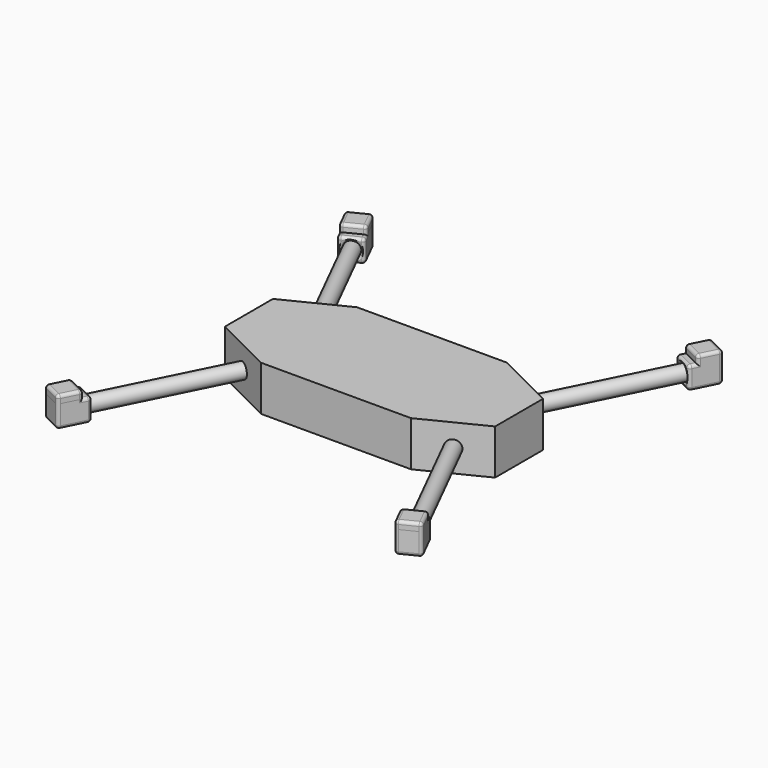
from build123d import *

# Parameters (mm, degrees)
F1_DEPTH      = 38.1
F2_R          = 6.35
F3_DEPTH      = 127
F4_W          = 19.05
F4_H          = 19.05
F5_DEPTH      = 12.7
F7_DEPTH      = 6.35
F9_T1_DEPTH   = 3.81
F9_T3_DEPTH   = 13.97
F9_T5_DEPTH   = 20.32
F9_T7_DEPTH   = 20.32
F9_T9_DEPTH   = 13.97
F9_T11_DEPTH  = 3.81
F9_T13_DEPTH  = 13.97
F9_T15_DEPTH  = 13.97
F9_T17_DEPTH  = 13.97
F9_S21_W      = 2.5908
F9_S21_H      = 2.5908
F9_T22_DEPTH  = 2.5908
F9_S27_W      = 2.5908
F9_S27_H      = 2.5908
F9_T28_DEPTH  = 2.5908
F9_S33_W      = 2.5908
F9_S33_H      = 2.5908
F9_T34_DEPTH  = 2.5908
F9_T40_DEPTH  = 2.5908
F9_S45_W      = 2.5908
F9_S45_H      = 2.5908
F9_T46_DEPTH  = 2.5908
F9_S51_W      = 2.5908
F9_S51_H      = 2.5908
F9_T52_DEPTH  = 2.5908
F9_S57_W      = 2.5908
F9_S57_H      = 2.5908
F9_T58_DEPTH  = 2.5908
F9_S63_W      = 2.5908
F9_S63_H      = 2.5908
F9_T64_DEPTH  = 2.5908
F9_S69_W      = 2.5908
F9_S69_H      = 2.5908
F9_T70_DEPTH  = 2.5908
F9_S75_W      = 2.5908
F9_S75_H      = 2.5908
F9_T76_DEPTH  = 2.5908
F9_T85_DEPTH  = 10.16
F9_T89_DEPTH  = 10.16
F9_T96_DEPTH  = 10.16
F9_T100_DEPTH = 10.16


# Not quite as in the source:
# - a fillet or chamfer that OpenCascade refuses, or shapes differently, is made with other operations: its cross-section is extruded or revolved along the edge and cut away or added


with BuildPart() as f1:
    # F0 (on Top) → F1 (new body)
    with BuildSketch(Plane.XY):
        Polygon((-63.5, 50.8), (-114.3, 25.4), (-114.3, -25.4), (-63.5, -50.8), (63.5, -50.8), (114.3, -25.4), (114.3, 25.4), (63.5, 50.8), align=None)
    extrude(amount=F1_DEPTH)


with BuildPart() as f3:
    # F2 (on face) → F3 (new body)
    with BuildSketch(Plane(origin=(-33.02, -66.04, 0), x_dir=(0.894427191, -0.4472135955, 0), z_dir=(-0.4472135955, -0.894427191, 0))):
        with Locations((-62.4757392913, 19.05)):
            Circle(F2_R)
    extrude(amount=F3_DEPTH)


with BuildPart() as f5:
    # F4 (on face) → F5 (new body, symmetric)
    with BuildSketch(Plane(origin=(-89.8161266285, -179.632253257, 0), x_dir=(0.894427191, -0.4472135955, 0), z_dir=(-0.4472135955, -0.894427191, 0))):
        with Locations((-62.4757392913, 19.05)):
            Rectangle(F4_W, F4_H)
    extrude(amount=F5_DEPTH, both=True)

    # F6 (on face) → F7 (join)
    with BuildSketch(Plane.XY.offset(28.575)):
        Polygon((-151.3757392913, -141.752931097), (-159.8951582856, -158.7917690856), (-142.8563202971, -167.3111880798), (-134.3369013028, -150.2723500913), align=None)
    extrude(amount=F7_DEPTH)

    # F8: cut F3
    add(f3.part, mode=Mode.SUBTRACT)

    # F9: fillet of radius 2.54 on 18 edges, made by hand

    # F9_s2 → F9_t1 (cut)
    with BuildSketch(Plane(origin=(-85.2724364982, -170.5448729964, 0), x_dir=(0, 0, 1), z_dir=(-0.4472135955, -0.894427191, 0))):
        with BuildLine():
            ThreePointArc((28.575, 69.4607392913), (27.8310512242, 71.2567905156), (26.035, 72.0007392913))
            Line((26.035, 72.0007392913), (28.575, 72.0007392913))
            Line((28.575, 72.0007392913), (28.575, 69.4607392913))
        make_face()
        with BuildLine():
            ThreePointArc((26.035, 52.9507392913), (27.8310512242, 53.6946880671), (28.575, 55.4907392913))
            Line((28.575, 55.4907392913), (28.575, 52.9507392913))
            Line((28.575, 52.9507392913), (26.035, 52.9507392913))
        make_face()
    extrude(amount=F9_T1_DEPTH, mode=Mode.SUBTRACT)

    # F9_s4 → F9_t3 (cut)
    with BuildSketch(Plane.XY.offset(12.065)):
        with BuildLine():
            ThreePointArc((-146.2640878948, -137.2092409667), (-148.203228953, -137.0714304548), (-149.6718554925, -138.3451634993))
            Line((-149.6718554925, -138.3451634993), (-148.5359329599, -136.0733184342))
            Line((-148.5359329599, -136.0733184342), (-146.2640878948, -137.2092409667))
        make_face()
        with BuildLine():
            ThreePointArc((-132.6330175039, -146.8645824936), (-132.495206992, -144.9254414353), (-133.7689400365, -143.4568148959))
            Line((-133.7689400365, -143.4568148959), (-131.4970949714, -144.5927374284))
            Line((-131.4970949714, -144.5927374284), (-132.6330175039, -146.8645824936))
        make_face()
    extrude(amount=F9_T3_DEPTH, mode=Mode.SUBTRACT)

    # F9_s6 → F9_t5 (cut)
    with BuildSketch(Plane(origin=(-94.3598167588, -188.7196335175, 0), x_dir=(0, 0, 1), z_dir=(0.4472135955, 0.894427191, 0))):
        with BuildLine():
            ThreePointArc((9.525, -69.4607392913), (10.2689487758, -71.2567905156), (12.065, -72.0007392913))
            Line((12.065, -72.0007392913), (9.525, -72.0007392913))
            Line((9.525, -72.0007392913), (9.525, -69.4607392913))
        make_face()
        with BuildLine():
            ThreePointArc((12.065, -52.9507392913), (10.2689487758, -53.6946880671), (9.525, -55.4907392913))
            Line((9.525, -55.4907392913), (9.525, -52.9507392913))
            Line((9.525, -52.9507392913), (12.065, -52.9507392913))
        make_face()
    extrude(amount=F9_T5_DEPTH, mode=Mode.SUBTRACT)

    # F9_s8 → F9_t7 (cut)
    with BuildSketch(Plane.XY.offset(12.065)):
        with BuildLine():
            ThreePointArc((-157.6233132205, -159.9276916181), (-158.897046265, -158.4590650787), (-158.759235753, -156.5199240204))
            Line((-158.759235753, -156.5199240204), (-159.8951582856, -158.7917690856))
            Line((-159.8951582856, -158.7917690856), (-157.6233132205, -159.9276916181))
        make_face()
        with BuildLine():
            ThreePointArc((-141.7203977645, -165.0393430147), (-143.189024304, -166.3130760592), (-145.1281653622, -166.1752655473))
            Line((-145.1281653622, -166.1752655473), (-142.8563202971, -167.3111880798))
            Line((-142.8563202971, -167.3111880798), (-141.7203977645, -165.0393430147))
        make_face()
    extrude(amount=F9_T7_DEPTH, mode=Mode.SUBTRACT)

    # F9_s10 → F9_t9 (cut)
    with BuildSketch(Plane(origin=(-88.1122428296, -176.2244856593, 0), x_dir=(0, 0, 1), z_dir=(-0.4472135955, -0.894427191, 0))):
        with BuildLine():
            ThreePointArc((34.925, 69.4607392913), (34.1810512242, 71.2567905156), (32.385, 72.0007392913))
            Line((32.385, 72.0007392913), (34.925, 72.0007392913))
            Line((34.925, 72.0007392913), (34.925, 69.4607392913))
        make_face()
    extrude(amount=F9_T9_DEPTH, mode=Mode.SUBTRACT)

    # F9_s12 → F9_t11 (cut)
    with BuildSketch(Plane.XY.offset(28.575)):
        with BuildLine():
            ThreePointArc((-149.1038942262, -142.8888536296), (-151.0430352845, -142.7510431177), (-152.5116618239, -144.0247761621))
            Line((-152.5116618239, -144.0247761621), (-151.3757392913, -141.752931097))
            Line((-151.3757392913, -141.752931097), (-149.1038942262, -142.8888536296))
        make_face()
        with BuildLine():
            ThreePointArc((-135.4728238354, -152.5441951564), (-135.3350133235, -150.6050540982), (-136.6087463679, -149.1364275587))
            Line((-136.6087463679, -149.1364275587), (-134.3369013028, -150.2723500913))
            Line((-134.3369013028, -150.2723500913), (-135.4728238354, -152.5441951564))
        make_face()
    extrude(amount=F9_T11_DEPTH, mode=Mode.SUBTRACT)

    # F9_s14 → F9_t13 (cut)
    with BuildSketch(Plane(origin=(-62.1275739291, 31.0637869646, 0), x_dir=(0, 0, 1), z_dir=(0.894427191, -0.4472135955, 0))):
        with BuildLine():
            ThreePointArc((34.925, 210.994964617), (34.1810512242, 212.7910158413), (32.385, 213.534964617))
            Line((32.385, 213.534964617), (34.925, 213.534964617))
            Line((34.925, 213.534964617), (34.925, 210.994964617))
        make_face()
        with BuildLine():
            ThreePointArc((12.065, 213.534964617), (10.2689487758, 212.7910158413), (9.525, 210.994964617))
            Line((9.525, 210.994964617), (9.525, 213.534964617))
            Line((9.525, 213.534964617), (12.065, 213.534964617))
        make_face()
        with BuildLine():
            ThreePointArc((12.065, 188.134964617), (10.2689487758, 188.8789133928), (9.525, 190.674964617))
            Line((9.525, 190.674964617), (9.525, 188.134964617))
            Line((9.525, 188.134964617), (12.065, 188.134964617))
        make_face()
    extrude(amount=F9_T13_DEPTH, mode=Mode.SUBTRACT)

    # F9_s16 → F9_t15 (cut)
    with BuildSketch(Plane(origin=(-94.3598167588, -188.7196335175, 0), x_dir=(0, 0, 1), z_dir=(0.4472135955, 0.894427191, 0))):
        with BuildLine():
            ThreePointArc((32.385, -52.9507392913), (34.1810512242, -53.6946880671), (34.925, -55.4907392913))
            Line((34.925, -55.4907392913), (34.925, -52.9507392913))
            Line((34.925, -52.9507392913), (32.385, -52.9507392913))
        make_face()
    extrude(amount=F9_T15_DEPTH, mode=Mode.SUBTRACT)

    # F9_s18 → F9_t17 (cut)
    with BuildSketch(Plane(origin=(-49.6324260709, 24.8162130354, 0), x_dir=(0, 0, 1), z_dir=(-0.894427191, 0.4472135955, 0))):
        with BuildLine():
            ThreePointArc((32.385, -194.484964617), (34.1810512242, -195.2289133928), (34.925, -197.024964617))
            Line((34.925, -197.024964617), (34.925, -194.484964617))
            Line((34.925, -194.484964617), (32.385, -194.484964617))
        make_face()
        with BuildLine():
            ThreePointArc((26.035, -188.134964617), (27.8310512242, -188.8789133928), (28.575, -190.674964617))
            Line((28.575, -190.674964617), (28.575, -188.134964617))
            Line((28.575, -188.134964617), (26.035, -188.134964617))
        make_face()
    extrude(amount=F9_T17_DEPTH, mode=Mode.SUBTRACT)


with BuildPart() as f9_tool20:
    # F9_s21 → F9_t22 (new body)
    with BuildSketch(Plane(origin=(-85.2724364982, -170.5448729964, 0), x_dir=(0, 0, 1), z_dir=(0.4472135955, 0.894427191, 0))):
        with Locations((27.3304, -70.7561392913)):
            Rectangle(F9_S21_W, F9_S21_H)
    extrude(amount=F9_T22_DEPTH)

    # F9_s23 → F9_t24 (revolve, cut)
    with BuildSketch(Plane(origin=(-147.4000104273, -139.4810860319, 26.035), x_dir=(0.632455532, -0.316227766, -0.7071067812), z_dir=(0.632455532, -0.316227766, 0.7071067812))):
        with BuildLine():
            ThreePointArc((0, -2.54), (2.54, 0), (0, 2.54))
            Line((0, 2.54), (0, -2.54))
        make_face()
    revolve(axis=Axis((-147.4000104273, -139.4810860319, 26.035), (0.4472135955, 0.894427191, 0)), mode=Mode.SUBTRACT)


with BuildPart() as f5_1:
    add(f5.part)

    # F9_t19: cut F9_tool20
    add(f9_tool20.part, mode=Mode.SUBTRACT)


with BuildPart() as f9_tool26:
    # F9_s27 → F9_t28 (new body)
    with BuildSketch(Plane(origin=(-85.2724364982, -170.5448729964, 0), x_dir=(0, 0, 1), z_dir=(0.4472135955, 0.894427191, 0))):
        with Locations((10.7696, -70.7561392913)):
            Rectangle(F9_S27_W, F9_S27_H)
    extrude(amount=F9_T28_DEPTH)

    # F9_s29 → F9_t30 (revolve, cut)
    with BuildSketch(Plane(origin=(-147.4000104273, -139.4810860319, 12.065), x_dir=(0.632455532, -0.316227766, 0.7071067812), z_dir=(-0.632455532, 0.316227766, 0.7071067812))):
        with BuildLine():
            ThreePointArc((0, -2.54), (2.54, 0), (0, 2.54))
            Line((0, 2.54), (0, -2.54))
        make_face()
    revolve(axis=Axis((-147.4000104273, -139.4810860319, 12.065), (0.4472135955, 0.894427191, 0)), mode=Mode.SUBTRACT)


with BuildPart() as f5_2:
    add(f5_1.part)

    # F9_t25: cut F9_tool26
    add(f9_tool26.part, mode=Mode.SUBTRACT)


with BuildPart() as f9_tool32:
    # F9_s33 → F9_t34 (new body)
    with BuildSketch(Plane(origin=(-94.3598167588, -188.7196335175, 0), x_dir=(0, 0, 1), z_dir=(-0.4472135955, -0.894427191, 0))):
        with Locations((10.7696, 70.7561392913)):
            Rectangle(F9_S33_W, F9_S33_H)
    extrude(amount=F9_T34_DEPTH)

    # F9_s35 → F9_t36 (revolve, cut)
    with BuildSketch(Plane(origin=(-156.4873906879, -157.655846553, 12.065), x_dir=(0.632455532, -0.316227766, 0.7071067812), z_dir=(0.632455532, -0.316227766, -0.7071067812))):
        with BuildLine():
            ThreePointArc((0, -2.54), (2.54, 0), (0, 2.54))
            Line((0, 2.54), (0, -2.54))
        make_face()
    revolve(axis=Axis((-156.4873906879, -157.655846553, 12.065), (-0.4472135955, -0.894427191, 0)), mode=Mode.SUBTRACT)


with BuildPart() as f5_3:
    add(f5_2.part)

    # F9_t31: cut F9_tool32
    add(f9_tool32.part, mode=Mode.SUBTRACT)


with BuildPart() as f9_tool38:
    # F9_s39 → F9_t40 (new body)
    with BuildSketch(Plane.XY.offset(32.385)):
        Polygon((-156.4873906879, -157.655846553), (-157.6460316711, -159.9731285194), (-159.9633136376, -158.8144875362), (-158.8046726544, -156.4972055698), align=None)
    extrude(amount=F9_T40_DEPTH)

    # F9_s41 → F9_t42 (revolve, cut)
    with BuildSketch(Plane(origin=(-156.4873906879, -157.655846553, 32.385), x_dir=(0.9486832981, 0.316227766, 0), z_dir=(0.316227766, -0.9486832981, 0))):
        with BuildLine():
            ThreePointArc((0, -2.54), (2.54, 0), (0, 2.54))
            Line((0, 2.54), (0, -2.54))
        make_face()
    revolve(axis=Axis((-156.4873906879, -157.655846553, 32.385), (0, 0, 1)), mode=Mode.SUBTRACT)


with BuildPart() as f5_4:
    add(f5_3.part)

    # F9_t37: cut F9_tool38
    add(f9_tool38.part, mode=Mode.SUBTRACT)


with BuildPart() as f9_tool44:
    # F9_s45 → F9_t46 (new body)
    with BuildSketch(Plane(origin=(-88.1122428296, -176.2244856593, 0), x_dir=(0, 0, 1), z_dir=(0.4472135955, 0.894427191, 0))):
        with Locations((33.6804, -70.7561392913)):
            Rectangle(F9_S45_W, F9_S45_H)
    extrude(amount=F9_T46_DEPTH)

    # F9_s47 → F9_t48 (revolve, cut)
    with BuildSketch(Plane(origin=(-150.2398167588, -145.1606986947, 32.385), x_dir=(0.632455532, -0.316227766, -0.7071067812), z_dir=(0.632455532, -0.316227766, 0.7071067812))):
        with BuildLine():
            ThreePointArc((0, -2.54), (2.54, 0), (0, 2.54))
            Line((0, 2.54), (0, -2.54))
        make_face()
    revolve(axis=Axis((-150.2398167588, -145.1606986947, 32.385), (0.4472135955, 0.894427191, 0)), mode=Mode.SUBTRACT)


with BuildPart() as f5_5:
    add(f5_4.part)

    # F9_t43: cut F9_tool44
    add(f9_tool44.part, mode=Mode.SUBTRACT)


with BuildPart() as f9_tool50:
    # F9_s51 → F9_t52 (new body)
    with BuildSketch(Plane(origin=(-49.6324260709, 24.8162130354, 0), x_dir=(0, 0, 1), z_dir=(0.894427191, -0.4472135955, 0))):
        with Locations((33.6804, 212.290364617)):
            Rectangle(F9_S51_W, F9_S51_H)
    extrude(amount=F9_T52_DEPTH)

    # F9_s53 → F9_t54 (revolve, cut)
    with BuildSketch(Plane(origin=(-143.9922428296, -163.9034204821, 32.385), x_dir=(0.316227766, 0.632455532, -0.7071067812), z_dir=(-0.316227766, -0.632455532, -0.7071067812))):
        with BuildLine():
            ThreePointArc((0, -2.54), (2.54, 0), (0, 2.54))
            Line((0, 2.54), (0, -2.54))
        make_face()
    revolve(axis=Axis((-143.9922428296, -163.9034204821, 32.385), (0.894427191, -0.4472135955, 0)), mode=Mode.SUBTRACT)


with BuildPart() as f5_6:
    add(f5_5.part)

    # F9_t49: cut F9_tool50
    add(f9_tool50.part, mode=Mode.SUBTRACT)


with BuildPart() as f9_tool56:
    # F9_s57 → F9_t58 (new body)
    with BuildSketch(Plane(origin=(-49.6324260709, 24.8162130354, 0), x_dir=(0, 0, 1), z_dir=(0.894427191, -0.4472135955, 0))):
        with Locations((33.6804, 195.729564617)):
            Rectangle(F9_S57_W, F9_S57_H)
    extrude(amount=F9_T58_DEPTH)

    # F9_s59 → F9_t60 (revolve, cut)
    with BuildSketch(Plane(origin=(-137.7446689005, -151.4082726238, 32.385), x_dir=(-0.316227766, -0.632455532, -0.7071067812), z_dir=(-0.316227766, -0.632455532, 0.7071067812))):
        with BuildLine():
            ThreePointArc((0, -2.54), (2.54, 0), (0, 2.54))
            Line((0, 2.54), (0, -2.54))
        make_face()
    revolve(axis=Axis((-137.7446689005, -151.4082726238, 32.385), (0.894427191, -0.4472135955, 0)), mode=Mode.SUBTRACT)


with BuildPart() as f5_7:
    add(f5_6.part)

    # F9_t55: cut F9_tool56
    add(f9_tool56.part, mode=Mode.SUBTRACT)


with BuildPart() as f9_tool62:
    # F9_s63 → F9_t64 (new body)
    with BuildSketch(Plane(origin=(-49.6324260709, 24.8162130354, 0), x_dir=(0, 0, 1), z_dir=(0.894427191, -0.4472135955, 0))):
        with Locations((10.7696, 189.379564617)):
            Rectangle(F9_S63_W, F9_S63_H)
    extrude(amount=F9_T64_DEPTH)

    # F9_s65 → F9_t66 (revolve, cut)
    with BuildSketch(Plane(origin=(-134.9048625691, -145.728659961, 12.065), x_dir=(-0.316227766, -0.632455532, 0.7071067812), z_dir=(0.316227766, 0.632455532, 0.7071067812))):
        with BuildLine():
            ThreePointArc((0, -2.54), (2.54, 0), (0, 2.54))
            Line((0, 2.54), (0, -2.54))
        make_face()
    revolve(axis=Axis((-134.9048625691, -145.728659961, 12.065), (0.894427191, -0.4472135955, 0)), mode=Mode.SUBTRACT)


with BuildPart() as f5_8:
    add(f5_7.part)

    # F9_t61: cut F9_tool62
    add(f9_tool62.part, mode=Mode.SUBTRACT)


with BuildPart() as f9_tool68:
    # F9_s69 → F9_t70 (new body)
    with BuildSketch(Plane(origin=(-49.6324260709, 24.8162130354, 0), x_dir=(0, 0, 1), z_dir=(0.894427191, -0.4472135955, 0))):
        with Locations((27.3304, 189.379564617)):
            Rectangle(F9_S69_W, F9_S69_H)
    extrude(amount=F9_T70_DEPTH)

    # F9_s71 → F9_t72 (revolve, cut)
    with BuildSketch(Plane(origin=(-134.9048625691, -145.728659961, 26.035), x_dir=(-0.316227766, -0.632455532, -0.7071067812), z_dir=(-0.316227766, -0.632455532, 0.7071067812))):
        with BuildLine():
            ThreePointArc((0, -2.54), (2.54, 0), (0, 2.54))
            Line((0, 2.54), (0, -2.54))
        make_face()
    revolve(axis=Axis((-134.9048625691, -145.728659961, 26.035), (0.894427191, -0.4472135955, 0)), mode=Mode.SUBTRACT)


with BuildPart() as f5_9:
    add(f5_8.part)

    # F9_t67: cut F9_tool68
    add(f9_tool68.part, mode=Mode.SUBTRACT)


with BuildPart() as f9_tool74:
    # F9_s75 → F9_t76 (new body)
    with BuildSketch(Plane(origin=(-49.6324260709, 24.8162130354, 0), x_dir=(0, 0, 1), z_dir=(0.894427191, -0.4472135955, 0))):
        with Locations((10.7696, 212.290364617)):
            Rectangle(F9_S75_W, F9_S75_H)
    extrude(amount=F9_T76_DEPTH)

    # F9_s77 → F9_t78 (revolve, cut)
    with BuildSketch(Plane(origin=(-143.9922428296, -163.9034204821, 12.065), x_dir=(0.316227766, 0.632455532, 0.7071067812), z_dir=(0.316227766, 0.632455532, -0.7071067812))):
        with BuildLine():
            ThreePointArc((0, -2.54), (2.54, 0), (0, 2.54))
            Line((0, 2.54), (0, -2.54))
        make_face()
    revolve(axis=Axis((-143.9922428296, -163.9034204821, 12.065), (0.894427191, -0.4472135955, 0)), mode=Mode.SUBTRACT)


with BuildPart() as f5_10:
    add(f5_9.part)

    # F9_t73: cut F9_tool74
    add(f9_tool74.part, mode=Mode.SUBTRACT)

    # F9_s79 → F9_t80 (revolve, cut)
    with BuildSketch(Plane.XY.offset(19.05)):
        with BuildLine():
            ThreePointArc((-132.0650562377, -144.3087567953), (-134.0041972959, -144.1709462834), (-135.4728238354, -145.4446793279))
            Line((-135.4728238354, -145.4446793279), (-134.3369013028, -143.1728342627))
            Line((-134.3369013028, -143.1728342627), (-132.0650562377, -144.3087567953))
        make_face()
    revolve(axis=Axis((-140.0165139656, -140.3330279313, 19.05), (0.4472135955, 0.894427191, 0)), mode=Mode.SUBTRACT)


with BuildPart() as f9_tool83:
    # F9_s84 → F9_t85 (new body)
    with BuildSketch(Plane(origin=(-85.2724364982, -170.5448729964, 0), x_dir=(0, 0, 1), z_dir=(-0.4472135955, -0.894427191, 0))):
        with BuildLine():
            ThreePointArc((28.575, 69.4607392913), (27.8310512242, 71.2567905156), (26.035, 72.0007392913))
            Line((26.035, 72.0007392913), (28.575, 72.0007392913))
            Line((28.575, 72.0007392913), (28.575, 69.4607392913))
        make_face()
    extrude(amount=F9_T85_DEPTH)

    split(bisect_by=Plane(origin=(-86.9763202971, -173.9526405941, 0), x_dir=(0, 0, 1), z_dir=(-0.4472135955, -0.894427191, 0)), keep=Keep.TOP)


with BuildPart() as f9_tool87:
    # F9_s88 → F9_t89 (new body)
    with BuildSketch(Plane.XY.offset(22.225)):
        with BuildLine():
            ThreePointArc((-149.1038942262, -142.8888536296), (-151.0430352845, -142.7510431177), (-152.5116618239, -144.0247761621))
            Line((-152.5116618239, -144.0247761621), (-151.3757392913, -141.752931097))
            Line((-151.3757392913, -141.752931097), (-149.1038942262, -142.8888536296))
        make_face()
    extrude(amount=F9_T89_DEPTH)

    split(bisect_by=Plane.XY.offset(28.575), keep=Keep.BOTTOM)


with BuildPart() as f9_tool83_1:
    add(f9_tool83.part)

    # F9_t91: intersect F9_tool87
    add(f9_tool87.part, mode=Mode.INTERSECT)


with BuildPart() as f5_11:
    add(f5_10.part)

    # F9_t81: cut F9_tool83
    add(f9_tool83_1.part, mode=Mode.SUBTRACT)


with BuildPart() as f9_tool94:
    # F9_s95 → F9_t96 (new body)
    with BuildSketch(Plane(origin=(-85.2724364982, -170.5448729964, 0), x_dir=(0, 0, 1), z_dir=(-0.4472135955, -0.894427191, 0))):
        with BuildLine():
            ThreePointArc((26.035, 52.9507392913), (27.8310512242, 53.6946880671), (28.575, 55.4907392913))
            Line((28.575, 55.4907392913), (28.575, 52.9507392913))
            Line((28.575, 52.9507392913), (26.035, 52.9507392913))
        make_face()
    extrude(amount=F9_T96_DEPTH)

    split(bisect_by=Plane(origin=(-86.9763202971, -173.9526405941, 0), x_dir=(0, 0, 1), z_dir=(-0.4472135955, -0.894427191, 0)), keep=Keep.TOP)


with BuildPart() as f9_tool98:
    # F9_s99 → F9_t100 (new body)
    with BuildSketch(Plane.XY.offset(22.225)):
        with BuildLine():
            ThreePointArc((-135.4728238354, -152.5441951564), (-135.3350133235, -150.6050540982), (-136.6087463679, -149.1364275587))
            Line((-136.6087463679, -149.1364275587), (-134.3369013028, -150.2723500913))
            Line((-134.3369013028, -150.2723500913), (-135.4728238354, -152.5441951564))
        make_face()
    extrude(amount=F9_T100_DEPTH)

    split(bisect_by=Plane.XY.offset(28.575), keep=Keep.BOTTOM)


with BuildPart() as f9_tool94_1:
    add(f9_tool94.part)

    # F9_t102: intersect F9_tool98
    add(f9_tool98.part, mode=Mode.INTERSECT)


with BuildPart() as f5_12:
    add(f5_11.part)

    # F9_t92: cut F9_tool94
    add(f9_tool94_1.part, mode=Mode.SUBTRACT)


with BuildPart() as f10_1:
    # F10: instance of F3
    add(f3.part.mirror(Plane.YZ))


with BuildPart() as f10_2:
    # F10: instance of F5
    add(f5_12.part.mirror(Plane.YZ))


with BuildPart() as f11_1:
    # F11: instance of F10_2
    add(f10_2.part.mirror(Plane.XZ))


with BuildPart() as f11_2:
    # F11: instance of F10_1
    add(f10_1.part.mirror(Plane.XZ))


with BuildPart() as f11_3:
    # F11: instance of F3
    add(f3.part.mirror(Plane.XZ))


with BuildPart() as f11_4:
    # F11: instance of F5
    add(f5_12.part.mirror(Plane.XZ))


solid = Compound([f1.part, f3.part, f5_12.part, f10_1.part, f10_2.part, f11_1.part, f11_2.part, f11_3.part, f11_4.part])
